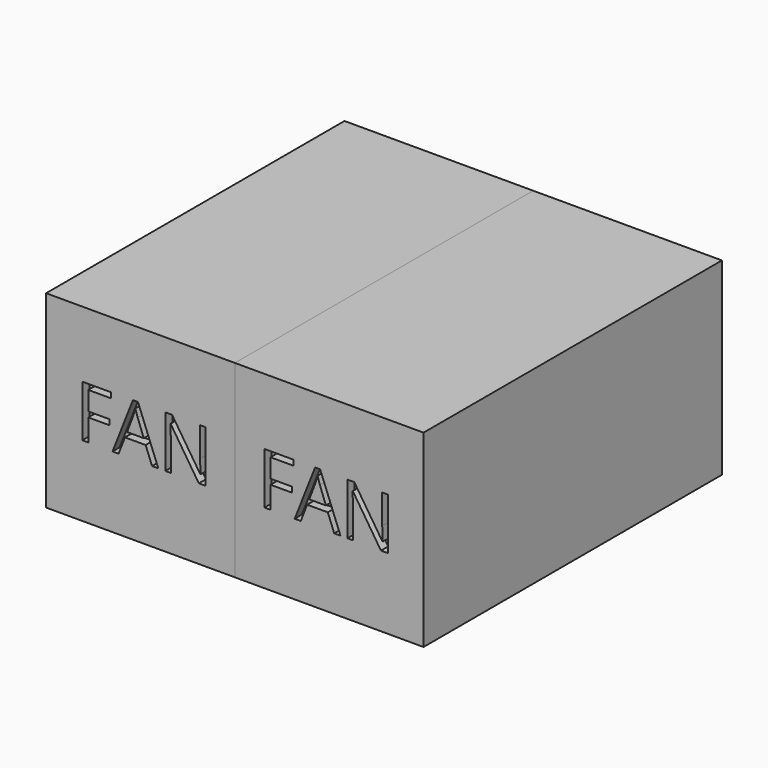
from build123d import *

# Parameters (mm, degrees)
F0_W         = 42
F0_H         = 42
F1_DEPTH     = 83
F2_R         = 1.5
F2_R_2       = 3
F3_DEPTH     = 25
F5_TEXT_SIZE = 16.0845695063
F6_DEPTH     = 2
F7_TEXT_SIZE = 16.0845695063
F8_DEPTH     = 2


# Not quite as in the source:
# - Text() gives the source's letters only with a copy of the font that has no kerning and outlines rounded to 1/6400 em; it was checked with that copy


with BuildPart() as f1:
    # F0 (on Front) → F1 (new body)
    with BuildSketch(Plane.XZ):
        with Locations((21, 21)):
            Rectangle(F0_W, F0_H)
    extrude(amount=F1_DEPTH)

    # F2 (on face) → F3 (cut)
    with BuildSketch(Plane(origin=(0, 0, 0), x_dir=(1, 0, 0), z_dir=(0, 0, -1))):
        with Locations((32, 50)):
            Circle(F2_R)
        with Locations((15, 50)):
            Circle(F2_R_2)
    extrude(amount=-F3_DEPTH, mode=Mode.SUBTRACT)


with BuildPart() as f4_1:
    # F4: instance of F1
    add(f1.part.mirror(Plane.YZ))

    # F7 (on face) → F8 (cut)
    with BuildSketch(Plane.XZ.offset(83)):
        with Locations((-35.5138107655, 15.8085655421)):
            Text('FAN', F7_TEXT_SIZE, font='Open Sans', text_align=(TextAlign.LEFT, TextAlign.BOTTOM))
    extrude(amount=-F8_DEPTH, mode=Mode.SUBTRACT)


with BuildPart() as f1_1:
    add(f1.part)

    # F5 (on face) → F6 (cut)
    with BuildSketch(Plane.XZ.offset(83)):
        with Locations((5.0263591111, 15.8085655421)):
            Text('FAN', F5_TEXT_SIZE, font='Open Sans', text_align=(TextAlign.LEFT, TextAlign.BOTTOM))
    extrude(amount=-F6_DEPTH, mode=Mode.SUBTRACT)


solid = Compound([f4_1.part, f1_1.part])
